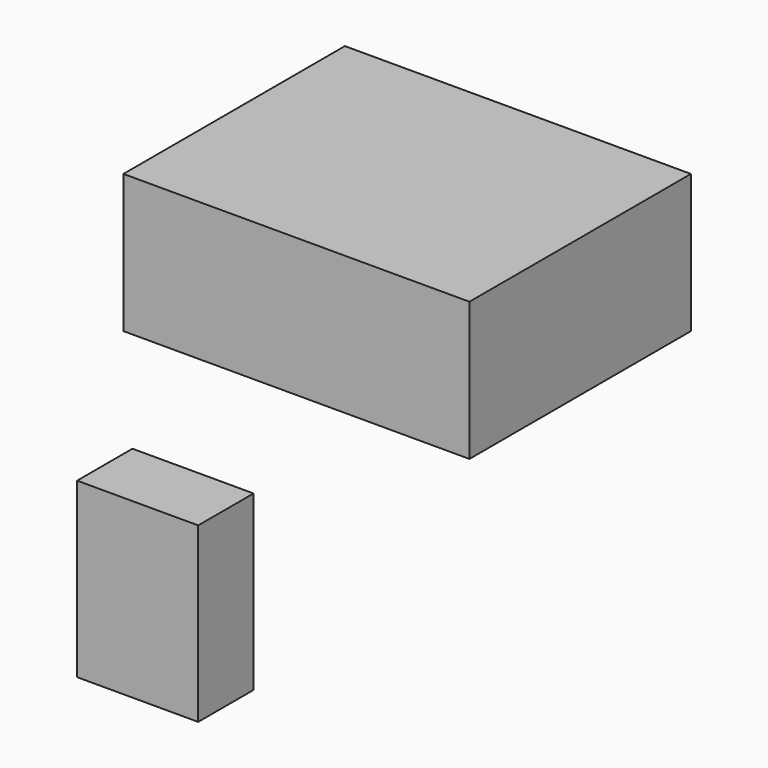
from build123d import *

# Parameters (mm, degrees)
F0_W     = 63.5
F0_H     = 50.8
F1_DEPTH = 25.4
F2_W     = 12.7
F2_H     = 31.75
F3_DEPTH = 22.225


# Not quite as in the source:
# - a length typed as a fraction of an inch, garbled in the dataset ("3 / 203.2 mm" for 3/8 in), is restored


with BuildPart() as f1:
    # F0 (on Top) → F1 (new body)
    with BuildSketch(Plane.XY):
        with Locations((-1.3241507113, 5.0739876905)):
            Rectangle(F0_W, F0_H)
    extrude(amount=F1_DEPTH)


with BuildPart() as f3:
    # F2 (on Right) → F3 (new body)
    with BuildSketch(Plane.YZ):
        with Locations((-65.9430525749, -8.1498604931)):
            Rectangle(F2_W, F2_H)
    extrude(amount=F3_DEPTH)


solid = Compound([f1.part, f3.part])
